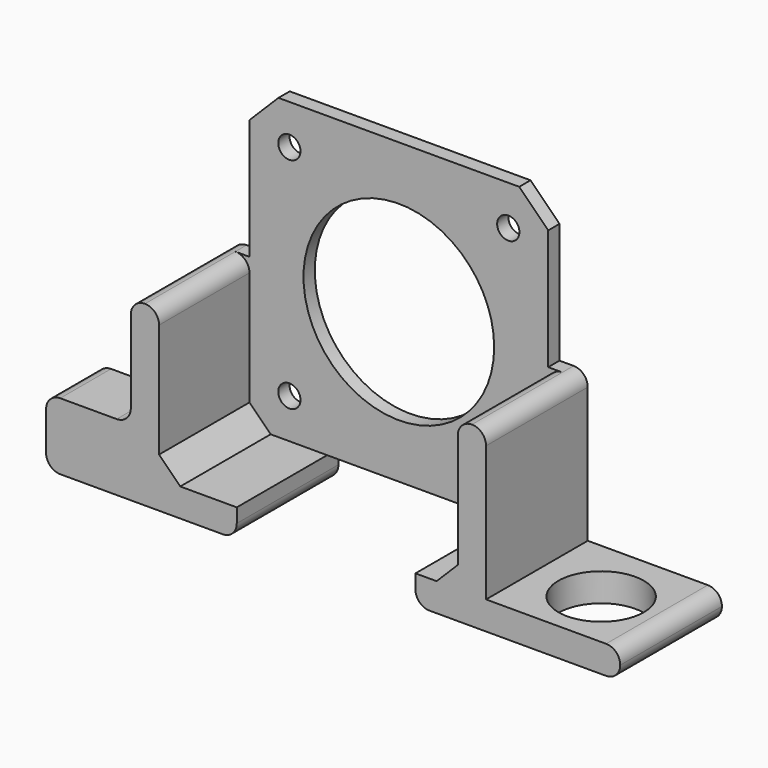
from build123d import *

# Parameters (mm, degrees)
F0_R     = 1.575
F0_R_2   = 13.5
F0_W     = 4
F0_H     = 21.15
F0_W_2   = 19
F0_H_2   = 4
F1_DEPTH = 2
F2_DEPTH = 18
F4_W     = 3
F4_H     = 9.4722927755
F4_W_2   = 9
F5_DEPTH = 12
F6_R     = 1.5
F7_DEPTH = 12.5
F3_R     = 6.05
F8_DEPTH = 25
F9_R     = 1.99999
F10_SIZE = 3


# Not quite as in the source:
# - a fillet or chamfer is up to 0.001 mm smaller than in the source, because OpenCascade refuses the exact size


with BuildPart() as f1:
    # F0 (on Front) → F1 (new body)
    with BuildSketch(Plane.XZ):
        Polygon((21.15, 17.0487806691), (17.0487806691, 21.15), (-17.0487806691, 21.15), (-21.15, 17.0487806691), (-21.15, 0), (-21.15, -21.15), (-10.15, -21.15), (15.15, -21.15), (21.15, -21.15), (21.15, 0), align=None)
        with Locations((-15.5, -15.5)):
            Circle(F0_R, mode=Mode.SUBTRACT)
        with Locations((15.5, -15.5)):
            Circle(F0_R, mode=Mode.SUBTRACT)
        Circle(F0_R_2, mode=Mode.SUBTRACT)
        with Locations((-15.5, 15.5)):
            Circle(F0_R, mode=Mode.SUBTRACT)
        with Locations((15.5, 15.5)):
            Circle(F0_R, mode=Mode.SUBTRACT)
        Polygon((-21.15, -21.15), (-21.15, 0), (-25.15, 0), (-25.15, -25.15), (-10.15, -25.15), (-10.15, -21.15), align=None)
        Polygon((25.15, -21.15), (21.15, -21.15), (15.15, -21.15), (15.15, -25.15), (25.15, -25.15), align=None)
        with Locations((23.15, -10.575)):
            Rectangle(F0_W, F0_H)
        with Locations((34.65, -23.15)):
            Rectangle(F0_W_2, F0_H_2)
    extrude(amount=F1_DEPTH)

    # F0 (on Front) → F2 (join)
    with BuildSketch(Plane.XZ):
        Polygon((-21.15, -21.15), (-21.15, 0), (-25.15, 0), (-25.15, -25.15), (-10.15, -25.15), (-10.15, -21.15), align=None)
        Polygon((25.15, -21.15), (21.15, -21.15), (15.15, -21.15), (15.15, -25.15), (25.15, -25.15), align=None)
        with Locations((34.65, -23.15)):
            Rectangle(F0_W_2, F0_H_2)
        with Locations((23.15, -10.575)):
            Rectangle(F0_W, F0_H)
    extrude(amount=F2_DEPTH)

    # F4 (on face) → F5 (join)
    with BuildSketch(Plane(origin=(-25.15, 0, 0), x_dir=(0, -1, 0), z_dir=(-1, 0, 0))):
        with Locations((1.5, -20.4138536122)):
            Rectangle(F4_W, F4_H)
        with Locations((13.5, -20.4138536122)):
            Rectangle(F4_W_2, F4_H)
    extrude(amount=F5_DEPTH)

    # F6 (on face) → F7 (cut, symmetric)
    with BuildSketch(Plane.XZ.offset(3)):
        with Locations((-34.15, -20.4138536122)):
            Circle(F6_R)
    extrude(amount=F7_DEPTH, both=True, mode=Mode.SUBTRACT)

    # F3 (on face) → F8 (cut)
    with BuildSketch(Plane.XY.offset(-21.15)):
        with Locations((34.65, -9.5)):
            Circle(F3_R)
    extrude(amount=-F8_DEPTH, mode=Mode.SUBTRACT)

    # F9 (radius 2 in the source; OpenCascade refuses exactly that, so slightly less here)
    f9_edges = [f1.edges().sort_by_distance(p)[0] for p in [
        (-25.15, -1.5, -15.677707),
        (-37.15, -1.5, -15.677707),
        (-37.15, -1.5, -25.15),
        (-37.15, -13.5, -15.677707),
        (-37.15, -13.5, -25.15),
        (-25.15, -13.5, -15.677707),
        (-10.15, -9, -25.15),
        (15.15, -9, -25.15),
        (44.15, -9, -25.15),
        (44.15, -9, -21.15),
        (25.15, -9, 0),
        (21.15, -10, 0),
        (-21.15, -10, 0),
        (-25.15, -9, 0),
    ]]
    fillet(f9_edges, radius=F9_R)

    # F10
    f10_edges = [f1.edges().sort_by_distance(p)[0] for p in [
        (21.15, -10, -21.15),
        (-21.15, -10, -21.15),
    ]]
    chamfer(f10_edges, length=F10_SIZE)


solid = f1.part
